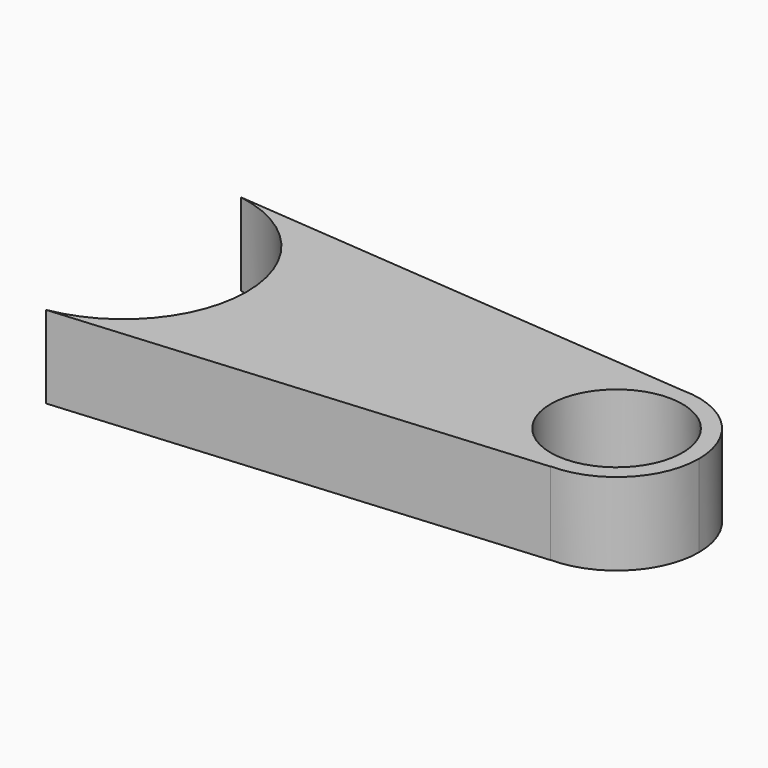
from build123d import *

# Parameters (mm, degrees)
F1_DEPTH = 5
F3_D     = 8


with BuildPart() as f1:
    # F0 (on Top) → F1 (new body)
    with BuildSketch(Plane.XY):
        with BuildLine():
            ThreePointArc((14.5967810947, -5), (18.1323150007, -3.5355339059), (19.5967810947, 0))
            ThreePointArc((19.5967810947, 0), (18.1323150007, 3.5355339059), (14.5967810947, 5))
            Line((14.5967810947, 5), (14.5967810947, 0))
            Line((14.5967810947, 0), (14.5967810947, -5))
        make_face()
        with BuildLine():
            Line((14.5967810947, 0), (14.5967810947, 5))
            ThreePointArc((14.5967810947, 5), (9.5967810947, 0), (14.5967810947, -5))
            Line((14.5967810947, -5), (14.5967810947, 0))
        make_face()
        with BuildLine():
            ThreePointArc((14.5967810947, -5), (9.5967810947, 0), (14.5967810947, 5))
            Line((14.5967810947, 5), (-14.1023044895, 7.3961588722))
            ThreePointArc((-14.1023044895, 7.3961588722), (-9.6198593647, 4.8436616619), (-7.8460222776, 0))
            ThreePointArc((-7.8460222776, 0), (-9.6226170145, -4.8469198667), (-14.110724196, -7.39756978))
            Line((-14.110724196, -7.39756978), (14.5967810947, -5.0171596368))
            Line((14.5967810947, -5.0171596368), (14.5967810947, -5))
        make_face()
    extrude(amount=F1_DEPTH)

    # F3 (through all)
    with Locations(Plane(origin=(0, 0, 0), x_dir=(1, 0, 0), z_dir=(0, 0, -1))):
        with Locations((14.5967810947, 0)):
            Hole(F3_D / 2)


solid = f1.part
